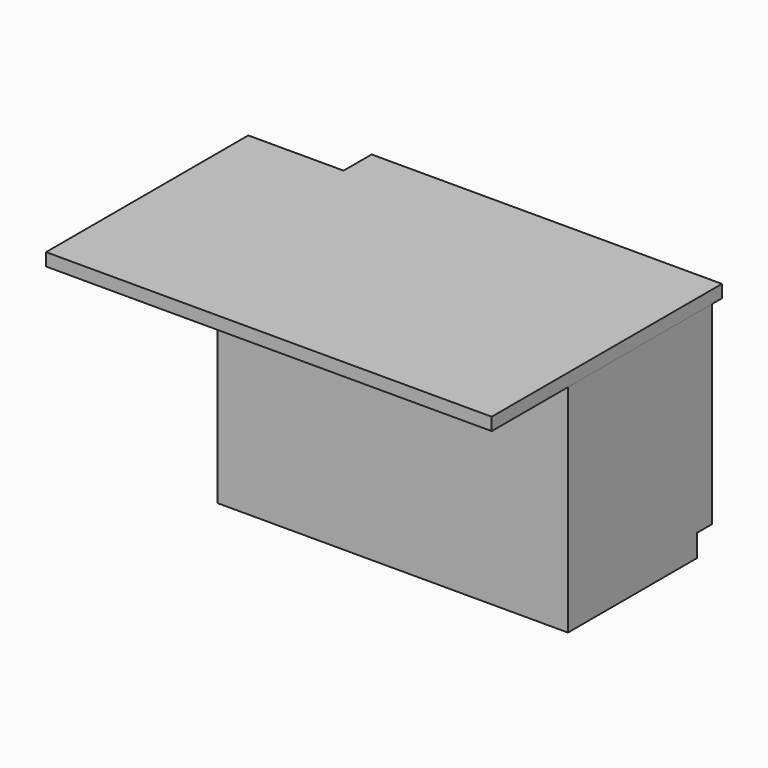
from build123d import *

# Parameters (mm, degrees)
F0_W     = 1400
F0_H     = 720
F1_DEPTH = 863.6
F2_W     = 76.2
F2_H     = 88.9
F3_DEPTH = 1400.001
F4_W     = 1150
F4_H     = 50.8
F5_DEPTH = 1400
F6_DEPTH = 381
F7_W     = 381
F7_H     = 140
F8_DEPTH = 50.8


with BuildPart() as f1:
    # F0 (on Top) → F1 (new body)
    with BuildSketch(Plane.XY):
        with Locations((700, 360)):
            Rectangle(F0_W, F0_H)
    extrude(amount=F1_DEPTH)

    # F2 (on Right) → F3 (cut, through all)
    with BuildSketch(Plane.YZ):
        with Locations((681.9, 44.45)):
            Rectangle(F2_W, F2_H)
    extrude(amount=F3_DEPTH, mode=Mode.SUBTRACT)


with BuildPart() as f5:
    # F4 (on Right) → F5 (new body, through all)
    with BuildSketch(Plane.YZ):
        with Locations((194, 889)):
            Rectangle(F4_W, F4_H)
    extrude(amount=F5_DEPTH)

    # F6 (add): a face of the model
    f6_faces = [f5.faces().sort_by_distance(p)[0] for p in [
        (0, 194, 889),
    ]]
    extrude(f6_faces, amount=F6_DEPTH)

    # F7 (on face) → F8 (cut, through all)
    with BuildSketch(Plane.XY.offset(914.4)):
        with Locations((-190.5, 699)):
            Rectangle(F7_W, F7_H)
    extrude(amount=-F8_DEPTH, mode=Mode.SUBTRACT)


solid = Compound([f1.part, f5.part])
